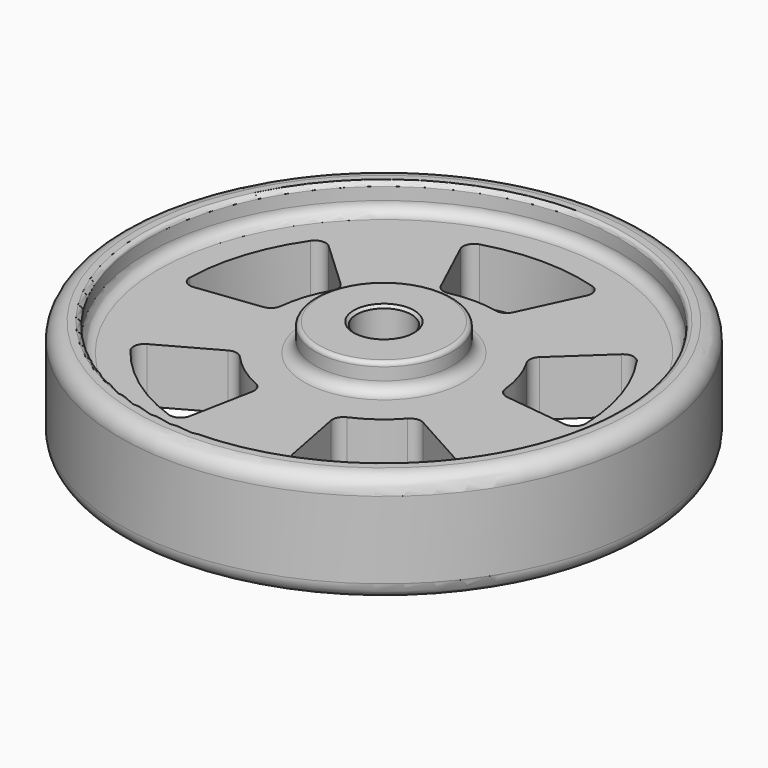
from build123d import *

# Parameters (mm, degrees)
F2_R            = 2
F3_R            = 3
F4_SIZE         = 0.5
F5_R            = 0.75
F8_DEPTH        = 20.001
F8_COPIES_COUNT = 5


# Not quite as in the source:
# - a pattern or mirror of a feature is missing from the dataset's text; its kind, count and spacing are read off the source's solid
# - a feature names something its author has since deleted; it is built from what else it names


with BuildPart() as f1:
    # F0 (on Front) → F1 (revolve)
    with BuildSketch(Plane.XZ):
        Polygon((-5, -20), (-5, 0), (-12.5, 0), (-12.5, -5), (-43, -5), (-43, 0), (-48, 0), (-48, -20), (-43, -20), (-43, -15), (-12.5, -15), (-12.5, -20), align=None)
    revolve(axis=Axis((0, 0, -8.972), (0, 0, -1)))

    # F2
    f2_edges = [f1.edges().sort_by_distance(p)[0] for p in [
        (12.5, 0, -5),
        (43, 0, -5),
        (12.5, 0, -15),
        (43, 0, -15),
    ]]
    fillet(f2_edges, radius=F2_R)

    # F3
    f3_edges = [f1.edges().sort_by_distance(p)[0] for p in [
        (48, 0, 0),
        (48, 0, -20),
    ]]
    fillet(f3_edges, radius=F3_R)

    # F4
    f4_edges = [f1.edges().sort_by_distance(p)[0] for p in [
        (12.5, 0, -20),
        (5, 0, -20),
        (5, 0, 0),
        (-5, 0, -10),
    ]]
    chamfer(f4_edges, length=F4_SIZE)

    # F5
    f5_edges = [f1.edges().sort_by_distance(p)[0] for p in [
        (-43, 0, -18.5),
        (43, 0, -17),
        (43, 0, -20),
        (-43, 0, -1.5),
        (43, 0, -3),
        (43, 0, 0),
        (12.5, 0, 0),
    ]]
    fillet(f5_edges, radius=F5_R)

    # F6 (on Top) → F8 (cut, through all)
    with BuildSketch(Plane.XY):
        with BuildLine():
            ThreePointArc((11.4938739259, 31.7472969271), (11.5050939944, 33.413279178), (10.2507441373, 34.5097413006))
            ThreePointArc((10.2507441373, 34.5097413006), (0, 36), (-10.2507441373, 34.5097413006))
            ThreePointArc((-10.2507441373, 34.5097413006), (-11.5050939944, 33.413279178), (-11.4938739259, 31.7472969271))
            Line((-11.4938739259, 31.7472969271), (-6.5522271295, 21.1499011734))
            ThreePointArc((-6.5522271295, 21.1499011734), (-5.629500751, 20.2040215031), (-4.3183127505, 20.040014346))
            ThreePointArc((-4.3183127505, 20.040014346), (0, 20.5), (4.3183127505, 20.040014346))
            ThreePointArc((4.3183127505, 20.040014346), (5.629500751, 20.2040215031), (6.5522271295, 21.1499011734))
            Line((6.5522271295, 21.1499011734), (11.4938739259, 31.7472969271))
        make_face()
    f8 = extrude(amount=-F8_DEPTH, mode=Mode.SUBTRACT)

    # F8_copies: F8 ×5 about axis
    f8_copies_axis = Axis((0, 0, 0), (0, 0, 1))
    for i in range(1, F8_COPIES_COUNT):
        add(f8.rotate(f8_copies_axis, i * 360 / F8_COPIES_COUNT), mode=Mode.SUBTRACT)


solid = f1.part
